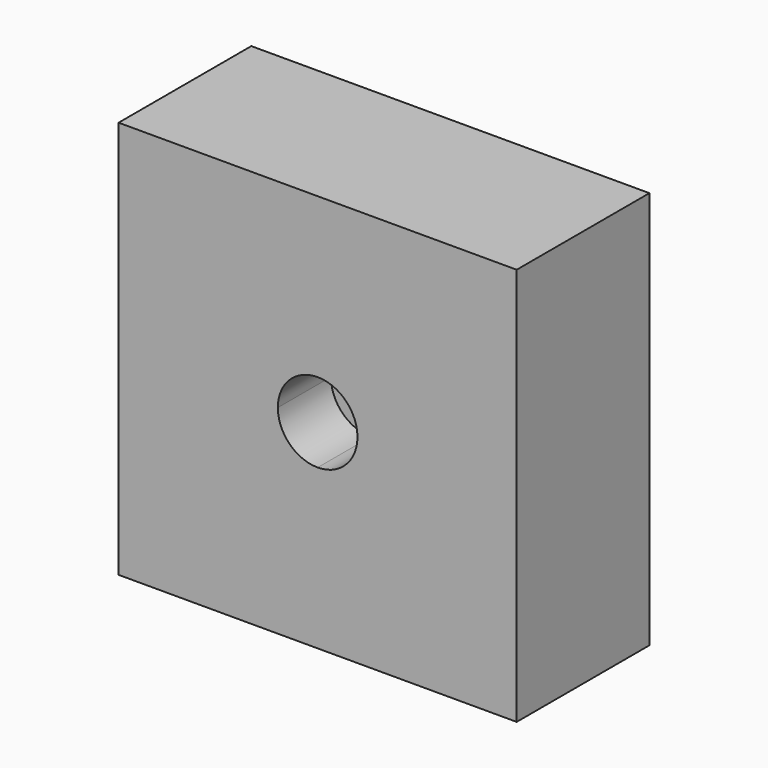
from build123d import *

# Parameters (mm, degrees)
F1_DEPTH = 25
F2_R     = 18.0741301682
F2_R_2   = 11.1620865302
F2_R_3   = 6
F3_DEPTH = 15


with BuildPart() as f1:
    # F0 (on Front) → F1 (new body)
    with BuildSketch(Plane.XZ):
        with BuildLine():
            ThreePointArc((-6, 0), (-4.2426406871, 4.2426406871), (0, 6))
            Line((0, 6), (0, 30))
            Line((0, 30), (-30, 30))
            Line((-30, 30), (-30, 0))
            Line((-30, 0), (-6, 0))
        make_face()
        with BuildLine():
            ThreePointArc((0, 6), (4.2426406871, 4.2426406871), (6, 0))
            Line((6, 0), (30, 0))
            Line((30, 0), (30, 30))
            Line((30, 30), (0, 30))
            Line((0, 30), (0, 6))
        make_face()
        with BuildLine():
            Line((30, 0), (6, 0))
            ThreePointArc((6, 0), (4.2426406871, -4.2426406871), (0, -6))
            Line((0, -6), (0, -30))
            Line((0, -30), (30, -30))
            Line((30, -30), (30, 0))
        make_face()
        with BuildLine():
            Line((0, -30), (0, -6))
            ThreePointArc((0, -6), (-4.2426406871, -4.2426406871), (-6, 0))
            Line((-6, 0), (-30, 0))
            Line((-30, 0), (-30, -30))
            Line((-30, -30), (0, -30))
        make_face()
    extrude(amount=F1_DEPTH)


with BuildPart() as f3:
    # F2 (on face) → F3 (new body)
    with BuildSketch(Plane(origin=(0, 0, 0), x_dir=(-1, 0, 0), z_dir=(0, 1, 0))):
        with Locations((0.5297824973, 0.1469794079)):
            Circle(F2_R)
        Circle(F2_R_2, mode=Mode.SUBTRACT)
        Circle(F2_R_2)
        Circle(F2_R_3, mode=Mode.SUBTRACT)
        Circle(F2_R_3)
    extrude(amount=-F3_DEPTH)


solid = Compound([f1.part, f3.part])
